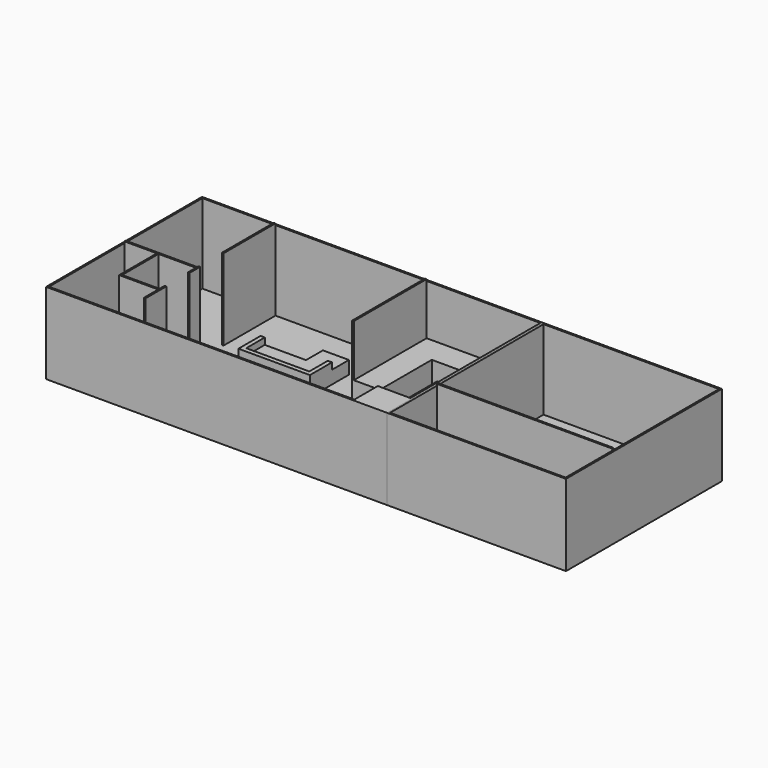
from build123d import *

# Parameters (mm, degrees)
F0_W         = 105000
F0_H         = 60000
F1_DEPTH     = 25000
F2_T         = -500
F3_W         = 500
F3_H         = 20000
F3_H_2       = 28000
F4_DEPTH     = 25000
F5_W         = 9000
F5_H         = 20000
F6_DEPTH     = 9000
F7_W         = 2000
F7_H         = 2000
F8_DEPTH     = 7000
F9_W         = 20000
F9_H         = 10000
F10_DEPTH    = 1000
F12_DEPTH    = 4000
F14_DEPTH    = 2000
F15_W        = 35000
F15_H        = 9000
F16_DEPTH    = 24500
F17_T4_DEPTH = 73292.0746991478
F18_W        = 55000
F18_H        = 60000
F19_DEPTH    = 25000
F20_T        = -500
F21_W        = 54000
F21_H        = 500
F22_DEPTH    = 25000


# Not quite as in the source:
# - a fillet or chamfer that OpenCascade refuses, or shapes differently, is made with other operations: its cross-section is extruded or revolved along the edge and cut away or added


with BuildPart() as f1:
    # F0 (on Top) → F1 (new body)
    with BuildSketch(Plane.XY):
        Rectangle(F0_W, F0_H)
    extrude(amount=F1_DEPTH)

    # F2
    f2_openings = [f1.faces().sort_by_distance(p)[0] for p in [
        (0, 0, 25000),
    ]]
    offset(amount=F2_T, openings=f2_openings)

    # F3 (on face) → F4 (join)
    with BuildSketch(Plane.XY.offset(500)):
        with Locations((-29750, 19500)):
            Rectangle(F3_W, F3_H)
        Polygon((-29500, -3500), (-29500, 500), (-30000, 500), (-30000, 0), (-52000, 0), (-52000, -500), (-42000, -500), (-42000, -15000), (-30000, -15000), (-30000, -20500), (-29500, -20500), (-29500, -12500), (-30000, -12500), (-30000, -14500), (-41500, -14500), (-41500, -500), (-30000, -500), (-30000, -3500), align=None)
        with Locations((16750, 15500)):
            Rectangle(F3_W, F3_H_2)
    extrude(amount=F4_DEPTH)

    # F5 (on face) → F6 (join)
    with BuildSketch(Plane.XY.offset(500)):
        Polygon((17000, 29500), (17000, 1500), (25000, 1500), (25000, 21500), (52000, 21500), (52000, 29500), align=None)
        with Locations((37500, 3500)):
            Rectangle(F5_W, F5_H)
    extrude(amount=F6_DEPTH)

    # F7 (on face) → F8 (join)
    with BuildSketch(Plane.XY.offset(500)):
        with Locations((-12000, -19500)):
            Rectangle(F7_W, F7_H)
        with Locations((-12000, -11500)):
            Rectangle(F7_W, F7_H)
        with Locations((6000, -11500)):
            Rectangle(F7_W, F7_H)
        with Locations((6000, -19500)):
            Rectangle(F7_W, F7_H)
    extrude(amount=F8_DEPTH)

    # F9 (on face) → F10 (join)
    with BuildSketch(Plane.XY.offset(7500)):
        with Locations((-3000, -15500)):
            Rectangle(F9_W, F9_H)
    extrude(amount=F10_DEPTH)

    # F11 (on face) → F12 (join)
    with BuildSketch(Plane.XY.offset(500)):
        Polygon((-4500, 10000), (-18500, 10000), (-18500, 1500), (3500, 1500), (3500, 16500), (-4500, 16500), align=None)
    extrude(amount=F12_DEPTH)

    # F13 (on face) → F14 (join)
    with BuildSketch(Plane.XY.offset(4500)):
        Polygon((-17200, 10000), (-18500, 10000), (-18500, 1500), (3500, 1500), (3500, 10000), (2200, 10000), (2200, 2881.0291290283), (-17200, 2881.0291290283), align=None)
    extrude(amount=F14_DEPTH)

    # F15 (on face) → F16 (join)
    with BuildSketch(Plane.XY.offset(500)):
        with Locations((34500, -25000)):
            Rectangle(F15_W, F15_H)
    extrude(amount=F16_DEPTH)

    # F17: chamfer of 25000 on 1 edges, made by hand


with BuildPart() as f17_tool2:
    # F17_s3 → F17_t4 (new body)
    with BuildSketch(Plane.XZ.offset(-43792.0746991478)):
        Polygon((42000, 25000), (17000, 0), (17000, 25000), align=None)
    extrude(amount=F17_T4_DEPTH)

    split(bisect_by=Plane.XY.offset(500), keep=Keep.TOP)

    split(bisect_by=Plane.XZ.offset(-1500), keep=Keep.TOP)


with BuildPart() as f1_1:
    add(f1.part)

    # F17_t1: cut F17_tool2
    add(f17_tool2.part, mode=Mode.SUBTRACT)


with BuildPart() as f19:
    # F18 (on Top) → F19 (new body)
    with BuildSketch(Plane.XY):
        with Locations((80000, 0)):
            Rectangle(F18_W, F18_H)
    extrude(amount=F19_DEPTH)

    # F20
    f20_openings = [f19.faces().sort_by_distance(p)[0] for p in [
        (80000, 0, 25000),
    ]]
    offset(amount=F20_T, openings=f20_openings)

    # F21 (on face) → F22 (join)
    with BuildSketch(Plane.XY.offset(500)):
        with Locations((80000, -11250)):
            Rectangle(F21_W, F21_H)
    extrude(amount=F22_DEPTH)


solid = Compound([f1_1.part, f19.part])
